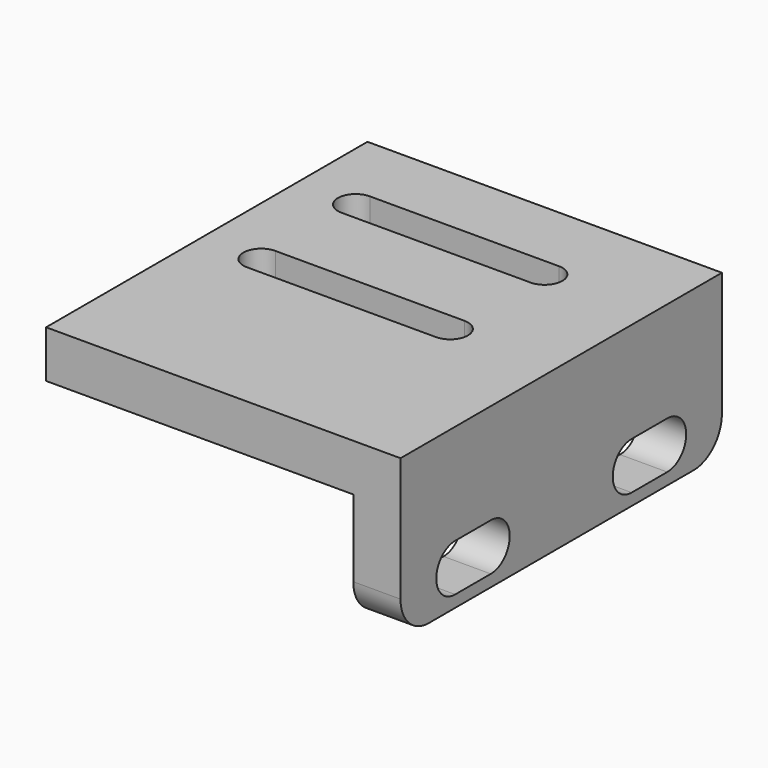
from build123d import *

# Parameters (mm, degrees)
F1_DEPTH = 4
F2_W     = 4
F2_H     = 34
F2_W_2   = 26
F3_DEPTH = 4


# Not quite as in the source:
# - a feature names something its author has since deleted; it is built from what else it names


with BuildPart() as f1:
    # F0 (on Right) → F1 (new body)
    with BuildSketch(Plane.YZ):
        with BuildLine():
            ThreePointArc((-3, 29.5474529266), (-2.1213203436, 31.6687732702), (0, 32.5474529266))
            Line((0, 32.5474529266), (28, 32.5474529266))
            ThreePointArc((28, 32.5474529266), (30.1213203436, 31.6687732702), (31, 29.5474529266))
            Line((31, 29.5474529266), (31, 36.0474529266))
            Line((31, 36.0474529266), (-3, 36.0474529266))
            Line((-3, 36.0474529266), (-3, 29.5474529266))
        make_face()
        with BuildLine():
            Line((28, 32.5474529266), (0, 32.5474529266))
            ThreePointArc((0, 32.5474529266), (-2.1213203436, 31.6687732702), (-3, 29.5474529266))
            ThreePointArc((-3, 29.5474529266), (-2.1213203436, 27.4261325831), (0, 26.5474529266))
            Line((0, 26.5474529266), (28, 26.5474529266))
            ThreePointArc((28, 26.5474529266), (30.1213203436, 27.4261325831), (31, 29.5474529266))
            ThreePointArc((31, 29.5474529266), (30.1213203436, 31.6687732702), (28, 32.5474529266))
        make_face()
        with BuildLine():
            ThreePointArc((2.7801140677, 27.5474529266), (0.7801140677, 29.5474529266), (2.7801140677, 31.5474529266))
            Line((2.7801140677, 31.5474529266), (6.5496175084, 31.5474529266))
            ThreePointArc((6.5496175084, 31.5474529266), (8.5496175084, 29.5474529266), (6.5496175084, 27.5474529266))
            Line((6.5496175084, 27.5474529266), (2.7801140677, 27.5474529266))
        make_face(mode=Mode.SUBTRACT)
        with BuildLine():
            Line((21.4503824916, 31.5474529266), (25.2198859323, 31.5474529266))
            ThreePointArc((25.2198859323, 31.5474529266), (27.2198859323, 29.5474529266), (25.2198859323, 27.5474529266))
            Line((25.2198859323, 27.5474529266), (21.4503824916, 27.5474529266))
            ThreePointArc((21.4503824916, 27.5474529266), (19.4503824916, 29.5474529266), (21.4503824916, 31.5474529266))
        make_face(mode=Mode.SUBTRACT)
    extrude(amount=-F1_DEPTH)

    # F2 (on face) → F3 (join)
    with BuildSketch(Plane.XY.offset(36.0474529266)):
        with Locations((-2, 14)):
            Rectangle(F2_W, F2_H)
        with Locations((-17, 14)):
            Rectangle(F2_W_2, F2_H)
        with BuildLine():
            ThreePointArc((-9, 15), (-7.5, 13.5), (-9, 12))
            Line((-9, 12), (-25, 12))
            ThreePointArc((-25, 12), (-26.5, 13.5), (-25, 15))
            Line((-25, 15), (-9, 15))
        make_face(mode=Mode.SUBTRACT)
        with BuildLine():
            ThreePointArc((-9, 25), (-7.5, 23.5), (-9, 22))
            Line((-9, 22), (-25, 22))
            ThreePointArc((-25, 22), (-26.5, 23.5), (-25, 25))
            Line((-25, 25), (-9, 25))
        make_face(mode=Mode.SUBTRACT)
    extrude(amount=F3_DEPTH)


solid = f1.part
